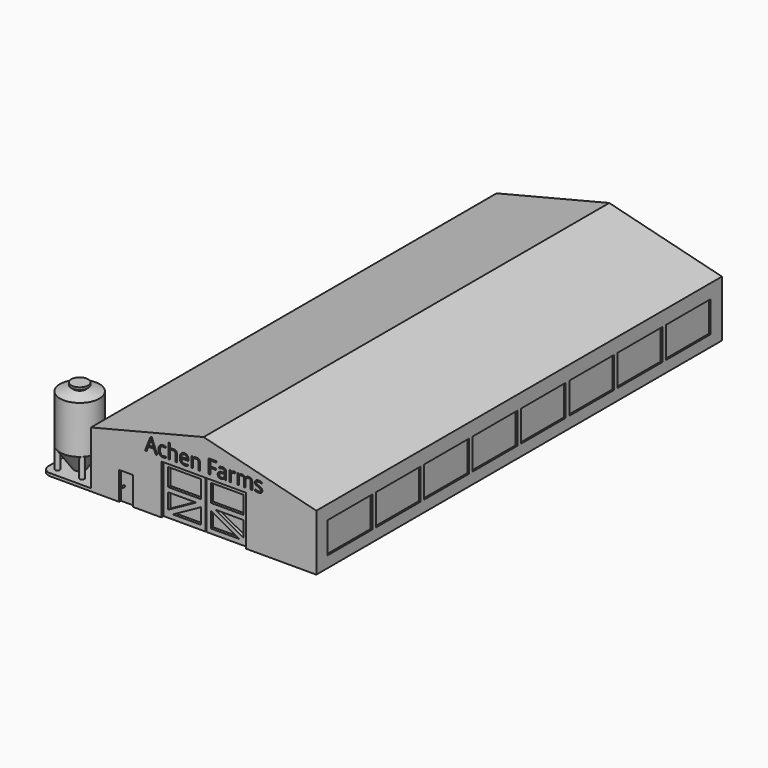
from build123d import *

# Parameters (mm, degrees)
F0_W          = 50.8
F0_H          = 12.7
F1_DEPTH      = 57.15
F2_W          = 19.05
F2_H          = 11.1125
F3_DEPTH      = 1.27
F5_DEPTH      = 0.635
F6_W          = 3.175
F6_H          = 6.35
F7_DEPTH      = 0.508
F8_R          = 0.1905
F9_DEPTH      = 0.508
F10_W         = 12.60475
F10_H         = 6.985
F11_DEPTH     = 0.381
F12_W         = 12.60475
F12_H         = 6.985
F13_DEPTH     = 0.381
F15_TEXT_SIZE = 4.4097222222
F16_DEPTH     = 0.381
F17_TEXT_SIZE = 4.4097222222
F18_DEPTH     = 0.381
F19_W         = 11.1125
F19_H         = 9.525
F20_DEPTH     = 0.635
F24_R         = 0.508
F25_DEPTH     = 12.7
F26_R         = 1.905


# Not quite as in the source:
# - a feature names something its author has since deleted; it is built from what else it names
# - Text() gives the source's letters only with a copy of the font that has no kerning and outlines rounded to 1/6400 em; it was checked with that copy


with BuildPart() as f1:
    # F0 (on Front) → F1 (new body)
    with BuildSketch(Plane.XZ):
        with Locations((0, 6.35)):
            Rectangle(F0_W, F0_H)
        Polygon((0, 19.05), (-25.4, 12.7), (25.4, 12.7), align=None)
    extrude(amount=F1_DEPTH)

    # F2 (on face) → F3 (cut)
    with BuildSketch(Plane.XZ.offset(57.15)):
        with Locations((0, 5.55625)):
            Rectangle(F2_W, F2_H)
    extrude(amount=-F3_DEPTH, mode=Mode.SUBTRACT)

    # F4 (on face) → F5 (join)
    with BuildSketch(Plane.XZ.offset(55.88)):
        Polygon((-9.525, 0), (-8.509, 0), (-8.509, 1.016), (-8.509, 1.5961883822), (-8.509, 5.08), (-8.509, 6.096), (-8.509, 10.0965), (-1.143, 10.0965), (-1.143, 6.096), (-1.143, 5.08), (-1.143, 4.4998116178), (-1.143, 1.016), (-1.143, 0), (-0.127, 0), (-0.127, 11.1125), (-9.525, 11.1125), align=None)
        Polygon((-2.1945914428, 5.08), (-1.143, 5.08), (-1.143, 6.096), (-8.509, 6.096), (-8.509, 5.08), align=None)
        Polygon((-8.509, 1.5961883822), (-8.509, 1.016), (-1.143, 5.08), (-2.1945914428, 5.08), align=None)
        Polygon((-1.143, 5.08), (-8.509, 1.016), (-7.4574085572, 1.016), (-1.143, 4.4998116178), align=None)
        Polygon((-8.509, 1.016), (-8.509, 0), (-1.143, 0), (-1.143, 1.016), (-7.4574085572, 1.016), align=None)
        Polygon((1.143, 1.016), (1.143, 0), (8.509, 0), (8.509, 1.016), (7.4574085572, 1.016), align=None)
        Polygon((0.127, 11.1125), (0.127, 0), (1.143, 0), (1.143, 1.016), (1.143, 4.4998116178), (1.143, 5.08), (1.143, 6.096), (1.143, 10.0965), (8.509, 10.0965), (8.509, 6.096), (8.509, 5.08), (8.509, 1.5961883822), (8.509, 1.016), (8.509, 0), (9.525, 0), (9.525, 11.1125), align=None)
        Polygon((1.143, 6.096), (1.143, 5.08), (2.1945914428, 5.08), (8.509, 5.08), (8.509, 6.096), align=None)
        Polygon((1.143, 5.08), (8.509, 1.016), (8.509, 1.5961883822), (2.1945914428, 5.08), align=None)
        Polygon((1.143, 5.08), (1.143, 4.4998116178), (7.4574085572, 1.016), (8.509, 1.016), align=None)
    extrude(amount=F5_DEPTH)

    # F6 (on face) → F7 (cut)
    with BuildSketch(Plane.XZ.offset(57.15)):
        with Locations((-17.4625, 3.175)):
            Rectangle(F6_W, F6_H)
    extrude(amount=-F7_DEPTH, mode=Mode.SUBTRACT)

    # F8 (on face) → F9 (join)
    with BuildSketch(Plane.XZ.offset(56.642)):
        with Locations((-18.288, 3.175)):
            Circle(F8_R)
    extrude(amount=F9_DEPTH)

    # F10 (on face) → F11 (cut)
    with BuildSketch(Plane(origin=(-25.4, 0, 0), x_dir=(0, -1, 0), z_dir=(-1, 0, 0))):
        with Locations((6.810375, 6.0325)):
            Rectangle(F10_W, F10_H)
        with Locations((20.431125, 6.0325)):
            Rectangle(F10_W, F10_H)
        with Locations((34.051875, 6.0325)):
            Rectangle(F10_W, F10_H)
        with Locations((47.672625, 6.0325)):
            Rectangle(F10_W, F10_H)
    extrude(amount=-F11_DEPTH, mode=Mode.SUBTRACT)

    # F12 (on face) → F13 (cut)
    with BuildSketch(Plane.YZ.offset(25.4)):
        with Locations((-47.672625, 6.0325)):
            Rectangle(F12_W, F12_H)
        with Locations((-34.051875, 6.0325)):
            Rectangle(F12_W, F12_H)
        with Locations((-20.431125, 6.0325)):
            Rectangle(F12_W, F12_H)
        with Locations((-6.810375, 6.0325)):
            Rectangle(F12_W, F12_H)
    extrude(amount=-F13_DEPTH, mode=Mode.SUBTRACT)

    # F14: F1 across plane


with BuildPart() as f1_1:
    add(f1.part)
    add(f1.part.mirror(Plane.XZ))

    # F15 (on face) → F16 (cut)
    with BuildSketch(Plane(origin=(0, 57.15, 0), x_dir=(-1, 0, 0), z_dir=(0, 1, 0))):
        with Locations((-13.2270996094, 12.065)):
            Text('Achen Farms', F15_TEXT_SIZE, font='Open Sans', text_align=(TextAlign.LEFT, TextAlign.BOTTOM))
    extrude(amount=-F16_DEPTH, mode=Mode.SUBTRACT)

    # F17 (on face) → F18 (cut)
    with BuildSketch(Plane.XZ.offset(57.15)):
        with Locations((-13.2270996094, 12.065)):
            Text('Achen Farms', F17_TEXT_SIZE, font='Open Sans', text_align=(TextAlign.LEFT, TextAlign.BOTTOM))
    extrude(amount=-F18_DEPTH, mode=Mode.SUBTRACT)

    # F19 (on face) → F20 (join)
    with BuildSketch(Plane(origin=(0, 0, 0), x_dir=(1, 0, 0), z_dir=(0, 0, -1))):
        with Locations((-30.95625, 52.3875)):
            Rectangle(F19_W, F19_H)
    extrude(amount=-F20_DEPTH)

    # F22 (on offset) → F23 (revolve)
    with BuildSketch(Plane.XZ.offset(52.3875)):
        Polygon((-36.195, 5.1693699214), (-33.02, 0.635), (-31.75, 0.635), (-31.75, 17.653), (-33.655, 17.653), (-33.655, 17.145), (-33.147, 17.145), (-33.147, 16.6917091385), (-36.195, 15.875), align=None)
    revolve(axis=Axis((-31.75, -52.3875, 9.144), (0, 0, 1)))

    # F24 (on face) → F25 (join)
    with BuildSketch(Plane.XY.offset(0.635)):
        with Locations((-34.5237218678, -55.1815)):
            Circle(F24_R)
        with Locations((-28.9762781322, -55.1815)):
            Circle(F24_R)
        with Locations((-34.5237218678, -49.5935)):
            Circle(F24_R)
        with Locations((-28.9762781322, -49.5935)):
            Circle(F24_R)
    extrude(amount=F25_DEPTH)

    # F26
    f26_edges = [f1_1.edges().sort_by_distance(p)[0] for p in [
        (-36.5125, -57.15, 0.3175),
        (-36.5125, -47.625, 0.3175),
    ]]
    fillet(f26_edges, radius=F26_R)


solid = f1_1.part
